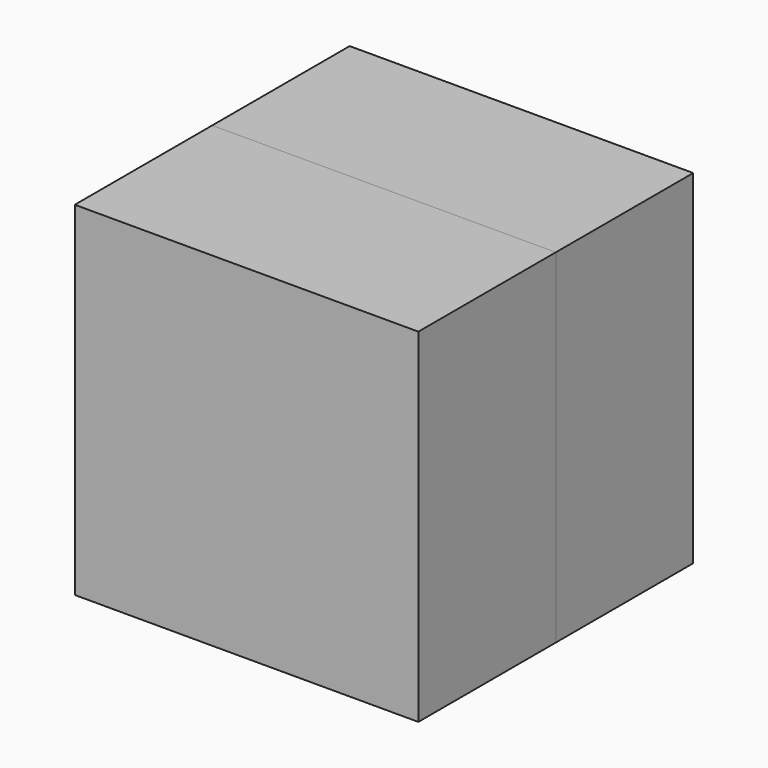
from build123d import *
from build123d import SkipClean  # not in build123d's __all__

# Parameters (mm, degrees)
F0_W     = 6
F0_H     = 6
F1_DEPTH = 3
F3_ANGLE = 180


with BuildPart() as f1:
    # F0 (on Front) → F1 (new body)
    with BuildSketch(Plane.XZ):
        with Locations((3.4017860889, -4.7885723032)):
            Rectangle(F0_W, F0_H)
    extrude(amount=F1_DEPTH)

    # F2 (on face) → F3 (revolve, cut)
    with BuildSketch(Plane.XZ.offset(3)):
        with BuildLine():
            ThreePointArc((3.4017860889, -6.7885723032), (5.4017860889, -4.7885723032), (3.4017860889, -2.7885723032))
            Line((3.4017860889, -2.7885723032), (3.4017860889, -6.7885723032))
        make_face()
    revolve(axis=Axis((3.4017860889, -3, -4.7885723032), (0, 0, 1)), revolution_arc=F3_ANGLE, mode=Mode.SUBTRACT)

    # F4: F1 across face


with BuildPart() as f1_1:
    add(f1.part, clean=False)
    with SkipClean():  # cleaning this boolean's faces spoils the solid; the shape is the same uncleaned
        add(f1.part.mirror(Plane(origin=(3.4017860889, -3, -4.7885723032), x_dir=(1, 0, 0), z_dir=(0, -1, 0))), clean=False)


solid = f1_1.part
